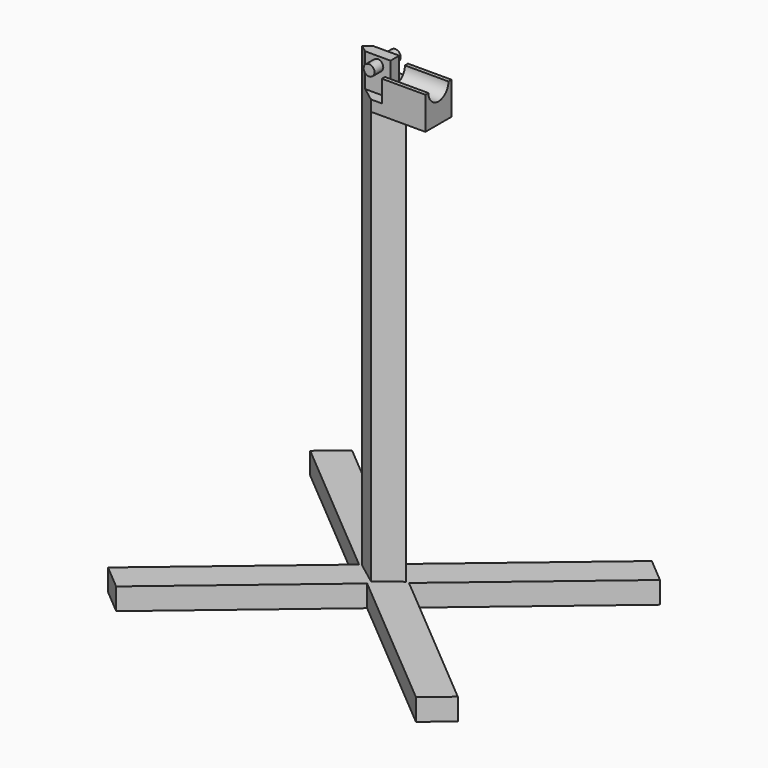
from build123d import *

# Parameters (mm, degrees)
F1_DEPTH       = 50.8
F3_DEPTH       = 1066.8
F5_DEPTH       = 26.67
F7_DEPTH       = 76.2
F8_R           = 29.21
F9_DEPTH       = 101.6
F11_DEPTH      = 0.366359725
F13_DEPTH      = 59.2676666667
F14_W          = 33.8666666667
F14_H          = 50.8
F14_W_2        = 25.4
F15_DEPTH      = 25.4
F16_W          = 33.8666666667
F16_H          = 26.3046402751
F16_W_2        = 25.4
F17_DEPTH      = 25.4
F18_R          = 12.7
F19_DEPTH      = 25.4
F19_DEPTH_BACK = 50.8


# Not quite as in the source:
# - a feature names something its author has since deleted; it is built from what else it names


with BuildPart() as f1:
    # F0 (on Top) → F1 (new body)
    with BuildSketch(Plane.XY):
        Polygon((-67.1887439802, 6.1155312845), (282.3736590158, -288.5672921234), (340.6340595151, -239.4534882221), (-8.9283434809, 55.2293351858), (340.6340595151, 349.9121585937), (282.3736590158, 399.025962495), (-67.1887439802, 104.3431390871), (-416.7511469763, 399.025962495), (-475.0115474756, 349.9121585937), (-125.4491444796, 55.2293351858), (-475.0115474756, -239.4534882221), (-416.7511469763, -288.5672921234), align=None)
    extrude(amount=-F1_DEPTH)

    # F2 (on face) → F3 (join)
    with BuildSketch(Plane.XY):
        Polygon((-67.1887439802, 93.3293351858), (-117.9887439802, 55.2293351858), (-67.1887439802, 17.1293351858), (-16.3887439802, 55.2293351858), align=None)
    extrude(amount=F3_DEPTH)

    # F4 (on face) → F5 (cut)
    with BuildSketch(Plane.XY.offset(1066.8)):
        Polygon((-67.1887439802, 17.1293351858), (-33.3220773136, 42.5293351858), (-101.0554106469, 42.5293351858), align=None)
        Polygon((-101.0554106469, 67.9293351858), (-33.3220773136, 67.9293351858), (-67.1887439802, 93.3293351858), align=None)
    extrude(amount=-F5_DEPTH, mode=Mode.SUBTRACT)

    # F6 (on face) → F7 (join)
    with BuildSketch(Plane.XY.offset(1040.13)):
        Polygon((59.8112560198, 93.3293351858), (-67.1887439802, 93.3293351858), (-33.3220773136, 67.9293351858), (-16.3887439802, 55.2293351858), (-33.3220773136, 42.5293351858), (-67.1887439802, 17.1293351858), (59.8112560198, 17.1293351858), align=None)
    extrude(amount=-F7_DEPTH)

    # F8 (on face) → F9 (cut)
    with BuildSketch(Plane.YZ.offset(59.8112560198)):
        with Locations((55.2293351858, 1040.13)):
            Circle(F8_R)
    extrude(amount=-F9_DEPTH, mode=Mode.SUBTRACT)

    # F10 (on face) → F11 (cut, through all)
    with BuildSketch(Plane.XY.offset(1066.8)):
        Polygon((-33.3220773136, 67.9293351858), (-41.7887439802, 67.9293351858), (-41.7887439802, 67.1429912157), (-32.2736186868, 67.1429912157), align=None)
        Polygon((-32.2736186868, 43.3156791558), (-41.7887439802, 43.3156791558), (-41.7887439802, 42.5293351858), (-33.3220773136, 42.5293351858), align=None)
    extrude(amount=-F11_DEPTH, mode=Mode.SUBTRACT)

    # F12 (on face) → F13 (cut, through all)
    with BuildSketch(Plane.YZ.offset(-41.7887439802)):
        with BuildLine():
            Line((42.5293351858, 1040.13), (26.0193351858, 1040.13))
            ThreePointArc((26.0193351858, 1040.13), (30.4887703175, 1024.601685539), (42.5293351858, 1013.8253597249))
            Line((42.5293351858, 1013.8253597249), (42.5293351858, 1040.13))
        make_face()
        with BuildLine():
            Line((84.4393351858, 1040.13), (67.9293351858, 1040.13))
            Line((67.9293351858, 1040.13), (67.9293351858, 1013.8253597249))
            ThreePointArc((67.9293351858, 1013.8253597249), (79.969900054, 1024.601685539), (84.4393351858, 1040.13))
        make_face()
    extrude(amount=-F13_DEPTH, mode=Mode.SUBTRACT)

    # F14 (on face) → F15 (cut)
    with BuildSketch(Plane.XZ.offset(-17.1293351858)):
        with Locations((-84.1220773136, 1014.73)):
            Rectangle(F14_W, F14_H)
        with Locations((-54.4887439802, 1014.73)):
            Rectangle(F14_W_2, F14_H)
    extrude(amount=-F15_DEPTH, mode=Mode.SUBTRACT)

    # F16 (on face) → F17 (cut)
    with BuildSketch(Plane(origin=(0, 93.3293351858, 0), x_dir=(-1, 0, 0), z_dir=(0, 1, 0))):
        with Locations((84.1220773136, 1026.9776798625)):
            Rectangle(F16_W, F16_H)
        with Locations((54.4887439802, 1026.9776798625)):
            Rectangle(F16_W_2, F16_H)
    extrude(amount=-F17_DEPTH, mode=Mode.SUBTRACT)

    # F18 (on face) → F19 (join, two sides)
    with BuildSketch(Plane.XZ.offset(-42.5293351858)) as f19_sk:
        with Locations((-71.4220773136, 1047.75)):
            Circle(F18_R)
    extrude(amount=F19_DEPTH)
    extrude(f19_sk.sketch, amount=-F19_DEPTH_BACK)


solid = f1.part
